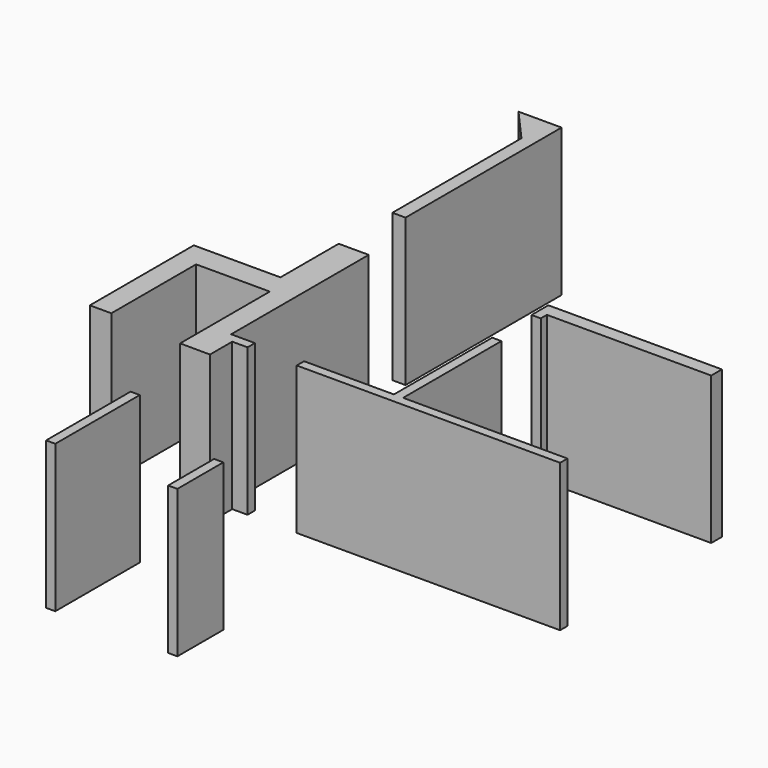
from build123d import *

# Parameters (mm, degrees)
F2_DEPTH = 2438.4
F0_W     = 152.4
F0_H     = 1746.8922138214
F0_H_2   = 950.3680467606


# Not quite as in the source:
# - the program builds the solid bodies; features that only make, move or delete a surface that nothing else refers to are left out


with BuildPart() as f2:
    # F0 (on Top) → F2 (new body)
    with BuildSketch(Plane.XY):
        Polygon((-3847.3440776825, 1188.7577511787), (-3847.3440776825, 1648.9702011108), (-3594.1724777222, 1648.9702011108), (-3594.1724777222, 1801.3702011108), (-3987.6942779541, 1801.3702011108), (-3987.6942779541, 4646.1702011108), (-4484.7030639648, 4646.1702011108), (-4484.7030639648, 3442.4197673798), (-5918.0942779541, 3442.4197673798), (-5918.0942779541, 3045.9702011108), (-5918.0942779541, 1293.3702011108), (-5562.4942779541, 1293.3702011108), (-5562.4942779541, 3045.9702011108), (-4343.2942779541, 3045.9702011108), (-4343.2942779541, 1191.7702011108), align=None)
    extrude(amount=F2_DEPTH)


with BuildPart() as f2b:
    # F0 (on Top) → F2, piece 2 (new body)
    with BuildSketch(Plane.XY):
        Polygon((-4267.0942779541, 5756.060754776), (-4267.0942779541, 8981.860754776), (-4979.4447412196, 8981.860754776), (-4484.7030639648, 8424.8667533997), (-4484.7030639648, 5930.2643890381), (-4484.7030639648, 5756.060754776), align=None)
    extrude(amount=F2_DEPTH)


with BuildPart() as f2c:
    # F0 (on Top) → F2, piece 3 (new body)
    with BuildSketch(Plane.XY):
        Polygon((-1142.8942779541, 4773.1702011108), (1574.9057220459, 4773.1702011108), (1574.9057220459, 4994.060754776), (-1295.2942779541, 4994.060754776), (-1295.2942779541, 4646.1702011108), (-1142.8942779541, 4646.1702011108), align=None)
    extrude(amount=F2_DEPTH)


with BuildPart() as f2d:
    # F0 (on Top) → F2, piece 4 (new body)
    with BuildSketch(Plane.XY):
        Polygon((-2781.3724777222, 1648.9702011108), (1574.9057220459, 1648.9702011108), (1574.9057220459, 1801.3702011108), (-1142.8942779541, 1801.3702011108), (-1142.8942779541, 3833.3702011108), (-1295.2942779541, 3833.3702011108), (-1295.2942779541, 1801.3702011108), (-2781.3724777222, 1801.3702011108), align=None)
    extrude(amount=F2_DEPTH)


with BuildPart() as f2e:
    # F0 (on Top) → F2, piece 5 (new body)
    with BuildSketch(Plane.XY):
        with Locations((-3923.5440776825, -1135.1836919785)):
            Rectangle(F0_W, F0_H)
    extrude(amount=F2_DEPTH)


with BuildPart() as f2f:
    # F0 (on Top) → F2, piece 6 (new body)
    with BuildSketch(Plane.XY):
        with Locations((-1904.8942779541, -1533.4457755089)):
            Rectangle(F0_W, F0_H_2)
    extrude(amount=F2_DEPTH)


solid = Compound([f2.part, f2b.part, f2c.part, f2d.part, f2e.part, f2f.part])
